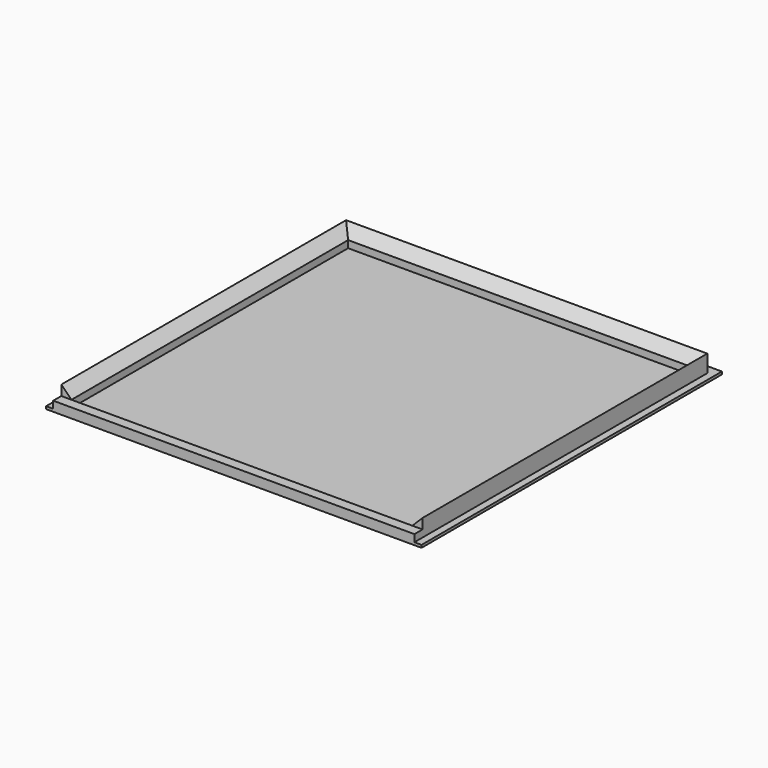
from build123d import *

# Parameters (mm, degrees)
F0_W         = 100
F0_H         = 100
F1_DEPTH     = 0.7
F2_W         = 96.2
F2_H         = 97.5
F2_W_2       = 90.8
F2_H_2       = 92.1
F3_DEPTH     = 1.9
F5_DEPTH     = 3
F6_T1_DEPTH  = 90.8
F6_T3_DEPTH  = 99.8150489639
F6_T9_DEPTH  = 99.8150489639
F6_T15_DEPTH = 98.5150489639
F6_T24_DEPTH = 99.8150489639
F6_T30_DEPTH = 98.5150489639


# Not quite as in the source:
# - a fillet or chamfer that OpenCascade refuses, or shapes differently, is made with other operations: its cross-section is extruded or revolved along the edge and cut away or added


with BuildPart() as f1:
    # F0 (on Top) → F1 (new body)
    with BuildSketch(Plane.XY):
        Rectangle(F0_W, F0_H)
    extrude(amount=F1_DEPTH)

    # F2 (on face) → F3 (join)
    with BuildSketch(Plane.XY.offset(0.7)):
        with Locations((0, -1.25)):
            Rectangle(F2_W, F2_H)
        with Locations((0, -1.25)):
            Rectangle(F2_W_2, F2_H_2, mode=Mode.SUBTRACT)
    extrude(amount=F3_DEPTH)

    # F4 (on face) → F5 (join)
    with BuildSketch(Plane.XY.offset(2.6)):
        Polygon((-48.1, -47.3), (-45.4, -47.3), (-45.4, 44.8), (45.4, 44.8), (45.4, -47.3), (48.1, -47.3), (48.1, 47.5), (-48.1, 47.5), align=None)
    extrude(amount=F5_DEPTH)

    # F6: chamfer of 3 on 3 edges, made by hand

    # F6_s2 → F6_t1 (cut)
    with BuildSketch(Plane.YZ.offset(-45.4)):
        Polygon((44.8, 2.6), (47.8, 5.6), (44.8, 5.6), align=None)
    extrude(amount=F6_T1_DEPTH, mode=Mode.SUBTRACT)

    # F6_s4 → F6_t3 (cut)
    with BuildSketch(Plane.XZ.offset(-44.8)):
        Polygon((-45.4, 2.6), (-48.4, 5.6), (-45.4, 5.6), align=None)
        Polygon((45.4, 2.6), (48.4, 5.6), (45.4, 5.6), align=None)
    extrude(amount=F6_T3_DEPTH, mode=Mode.SUBTRACT)


with BuildPart() as f6_tool7:
    # F6_s8 → F6_t9 (new body)
    with BuildSketch(Plane.XZ.offset(47.3)):
        Polygon((-45.4, 2.6), (-48.4, 5.6), (-45.4, 5.6), align=None)
    extrude(amount=-F6_T9_DEPTH)

    split(bisect_by=Plane.YZ.offset(-48.1), keep=Keep.TOP)

    split(bisect_by=Plane.XZ.offset(-44.8), keep=Keep.BOTTOM)

    split(bisect_by=Plane.XZ.offset(-47.5), keep=Keep.TOP)


with BuildPart() as f6_tool13:
    # F6_s14 → F6_t15 (new body)
    with BuildSketch(Plane.YZ.offset(-53.1150489639)):
        Polygon((44.8, 2.6), (47.8, 5.6), (44.8, 5.6), align=None)
    extrude(amount=F6_T15_DEPTH)

    split(bisect_by=Plane.YZ.offset(-48.1), keep=Keep.TOP)

    split(bisect_by=Plane.YZ.offset(-45.4), keep=Keep.BOTTOM)

    split(bisect_by=Plane.XZ.offset(-47.5), keep=Keep.TOP)


with BuildPart() as f6_tool7_1:
    add(f6_tool7.part)

    # F6_t19: intersect F6_tool13
    add(f6_tool13.part, mode=Mode.INTERSECT)


with BuildPart() as f1_1:
    add(f1.part)

    # F6_t5: cut F6_tool7
    add(f6_tool7_1.part, mode=Mode.SUBTRACT)


with BuildPart() as f6_tool22:
    # F6_s23 → F6_t24 (new body)
    with BuildSketch(Plane.XZ.offset(-52.5150489639)):
        Polygon((45.4, 2.6), (48.4, 5.6), (45.4, 5.6), align=None)
    extrude(amount=F6_T24_DEPTH)

    split(bisect_by=Plane.XZ.offset(-44.8), keep=Keep.BOTTOM)

    split(bisect_by=Plane.XZ.offset(-47.5), keep=Keep.TOP)

    split(bisect_by=Plane.YZ.offset(48.1), keep=Keep.BOTTOM)


with BuildPart() as f6_tool28:
    # F6_s29 → F6_t30 (new body)
    with BuildSketch(Plane.YZ.offset(-45.4)):
        Polygon((44.8, 2.6), (47.8, 5.6), (44.8, 5.6), align=None)
    extrude(amount=F6_T30_DEPTH)

    split(bisect_by=Plane.YZ.offset(45.4), keep=Keep.TOP)

    split(bisect_by=Plane.XZ.offset(-47.5), keep=Keep.TOP)

    split(bisect_by=Plane.YZ.offset(48.1), keep=Keep.BOTTOM)


with BuildPart() as f6_tool22_1:
    add(f6_tool22.part)

    # F6_t34: intersect F6_tool28
    add(f6_tool28.part, mode=Mode.INTERSECT)


with BuildPart() as f1_2:
    add(f1_1.part)

    # F6_t20: cut F6_tool22
    add(f6_tool22_1.part, mode=Mode.SUBTRACT)


solid = f1_2.part
